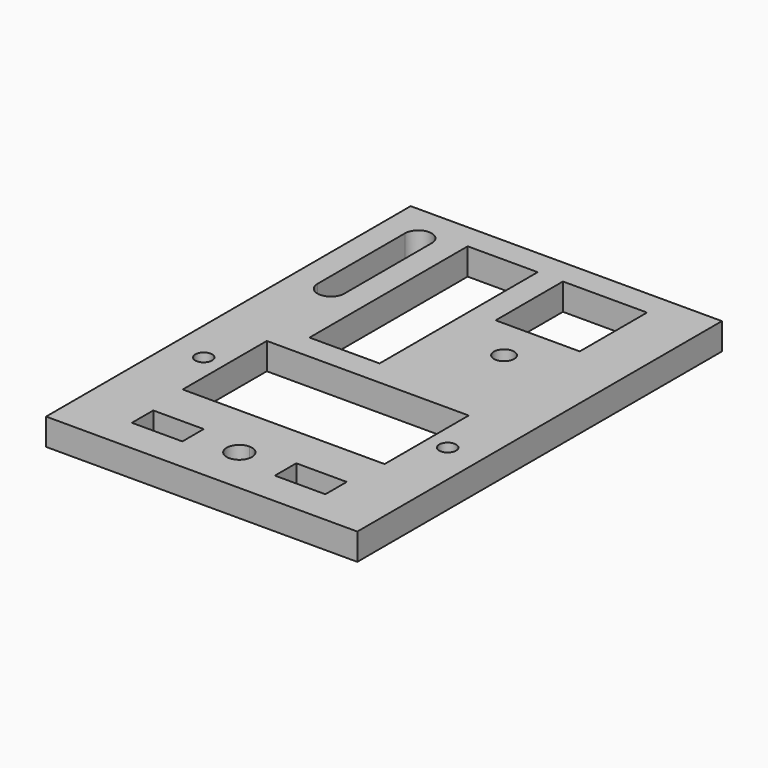
from build123d import *

# Parameters (mm, degrees)
F0_W     = 37
F0_H     = 54.175
F0_W_2   = 6
F0_H_2   = 3.175
F0_R     = 1
F0_W_3   = 8.325
F0_H_3   = 23.5
F0_W_4   = 10
F0_H_4   = 10
F0_R_2   = 1.2
F1_DEPTH = 3.175


# Not quite as in the source:
# - a length typed as a fraction of an inch, garbled in the dataset ("3 / 203.2 mm" for 3/8 in), is restored
# - a feature names something its author has since deleted; it is built from what else it names


with BuildPart() as f1:
    # F0 (on Top) → F1 (new body)
    with BuildSketch(Plane.XY):
        with Locations((13.6980720539, 20.2328219792)):
            Rectangle(F0_W, F0_H)
        with Locations((5.1980720539, -1.2671780208)):
            Rectangle(F0_W_2, F0_H_2, mode=Mode.SUBTRACT)
        with Locations((-0.8019279461, 11.5703219792)):
            Circle(F0_R, mode=Mode.SUBTRACT)
        with BuildLine():
            ThreePointArc((13.6980720539, 0.2328219792), (14.7587322257, -0.2065178491), (15.1980720539, -1.2671780208))
            ThreePointArc((15.1980720539, -1.2671780208), (12.6374118822, -2.3278381926), (13.6980720539, 0.2328219792))
        make_face(mode=Mode.SUBTRACT)
        with Locations((22.1980720539, -1.2671780208)):
            Rectangle(F0_W_2, F0_H_2, mode=Mode.SUBTRACT)
        Polygon((1.6980720539, 5.3203219792), (1.6980720539, 17.8203219792), (13.6980720539, 17.8203219792), (25.6980720539, 17.8203219792), (25.6980720539, 5.3203219792), align=None, mode=Mode.SUBTRACT)
        with Locations((28.1980720539, 11.5703219792)):
            Circle(F0_R, mode=Mode.SUBTRACT)
        with Locations((8.5355720539, 32.5703219792)):
            Rectangle(F0_W_3, F0_H_3, mode=Mode.SUBTRACT)
        with BuildLine():
            ThreePointArc((-1.8019279461, 42.7328219792), (-0.2144279461, 44.3203219792), (1.3730720539, 42.7328219792))
            Line((1.3730720539, 42.7328219792), (1.3730720539, 29.7328219792))
            ThreePointArc((1.3730720539, 29.7328219792), (-0.2144279461, 28.1453219792), (-1.8019279461, 29.7328219792))
            Line((-1.8019279461, 29.7328219792), (-1.8019279461, 42.7328219792))
        make_face(mode=Mode.SUBTRACT)
        Polygon((15.6980720539, 24.3203219792), (15.6980720539, 34.3203219792), (15.6980720539, 44.3203219792), (25.6980720539, 44.3203219792), (25.6980720539, 34.3203219792), (25.6980720539, 24.3203219792), align=None, mode=Mode.SUBTRACT)
        with Locations((20.6980720539, 29.3203219792)):
            Rectangle(F0_W_4, F0_H_4)
        with Locations((20.6980720539, 29.3203219792)):
            Circle(F0_R_2, mode=Mode.SUBTRACT)
    extrude(amount=F1_DEPTH)


solid = f1.part
